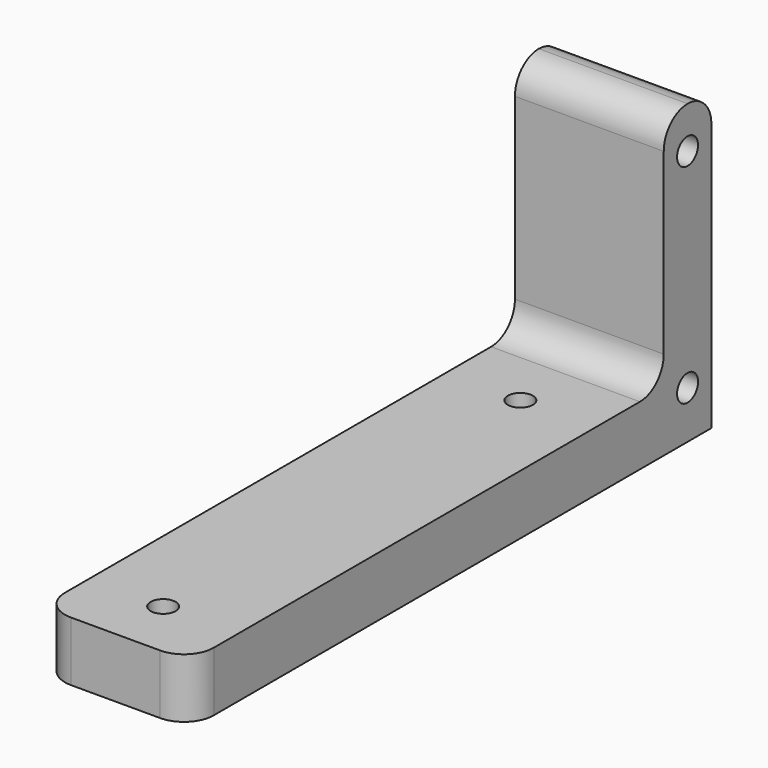
from build123d import *

# Parameters (mm, degrees)
F1_DEPTH = 25
F3_R     = 2.1
F4_DEPTH = 25
F6_R     = 2.2
F7_DEPTH = 25
F8_R     = 4.99999


# Not quite as in the source:
# - a fillet or chamfer is up to 0.001 mm smaller than in the source, because OpenCascade refuses the exact size


with BuildPart() as f1:
    # F0 (on Right) → F1 (new body)
    with BuildSketch(Plane.YZ):
        Polygon((-127.7586124506, 10), (-127.7586124506, 0), (-18.2758603601, 0), (-18.2758603601, 50), (-28.2758603601, 50), (-28.2758603601, 10), align=None)
    extrude(amount=F1_DEPTH)

    # F3 (on face) → F4 (cut)
    with BuildSketch(Plane.XY.offset(10)):
        with Locations((12.5, -117.7586124506)):
            Circle(F3_R)
        with Locations((12.5, -42.7586124506)):
            Circle(F3_R)
    extrude(amount=-F4_DEPTH, mode=Mode.SUBTRACT)

    # F6 (on face) → F7 (cut)
    with BuildSketch(Plane.YZ.offset(25)):
        with Locations((-23.2758603601, 43)):
            Circle(F6_R)
        with Locations((-23.2758603601, 8)):
            Circle(F6_R)
    extrude(amount=-F7_DEPTH, mode=Mode.SUBTRACT)

    # F8 (radius 5 in the source; OpenCascade refuses exactly that, so slightly less here)
    f8_edges = [f1.edges().sort_by_distance(p)[0] for p in [
        (12.5, -28.27586, 10),
        (12.5, -18.27586, 50),
        (12.5, -28.27586, 50),
        (25, -127.758612, 5),
        (0, -127.758612, 5),
    ]]
    fillet(f8_edges, radius=F8_R)


solid = f1.part
